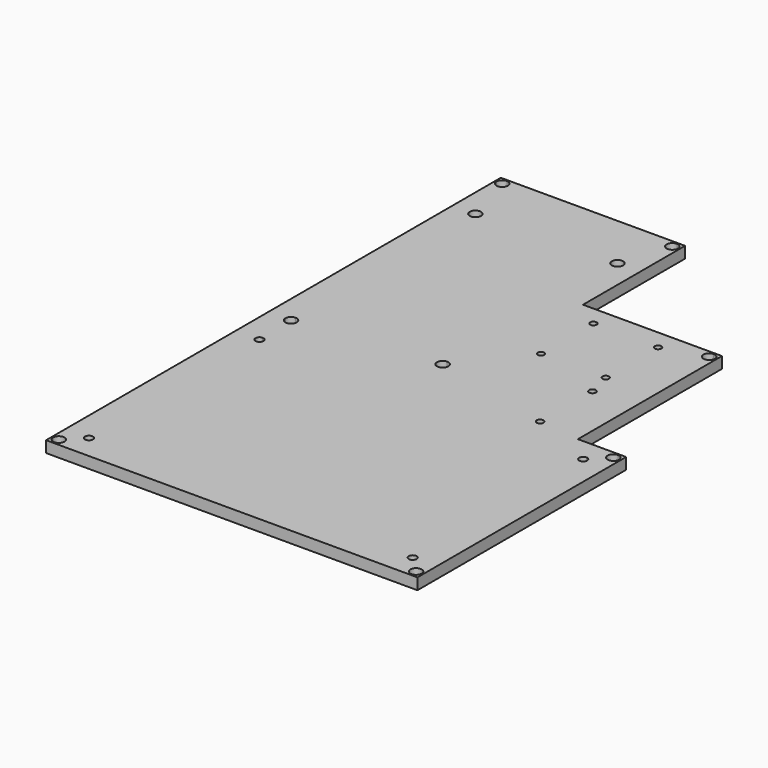
from build123d import *

# Parameters (mm, degrees)
F0_W     = 10
F0_H     = 17
F0_W_2   = 5
F0_H_2   = 5
F1_DEPTH = 4


with BuildPart() as f1:
    # F0 (on Top) → F1 (new body)
    with BuildSketch(Plane.XY):
        with BuildLine():
            Line((-37.7009056807, -58.8260023594), (-40.7009056807, -58.8260023594))
            Line((-40.7009056807, -58.8260023594), (-40.7009056807, -52.8260023594))
            Line((-40.7009056807, -52.8260023594), (-40.7009056807, 28.4739976406))
            Line((-40.7009056807, 28.4739976406), (-40.7009056807, 44.6739976406))
            Line((-40.7009056807, 44.6739976406), (14.2990943193, 44.6739976406))
            Line((14.2990943193, 44.6739976406), (14.2990943193, 49.6739976406))
            Line((14.2990943193, 49.6739976406), (-43.2009056807, 49.6739976406))
            Line((-43.2009056807, 49.6739976406), (-43.2009056807, 49.1739976406))
            ThreePointArc((-43.2009056807, 49.1739976406), (-41.7866921183, 48.588211203), (-41.2009056807, 47.1739976406))
            ThreePointArc((-41.2009056807, 47.1739976406), (-43.2009056807, 45.1739976406), (-45.2009056807, 47.1739976406))
            Line((-45.2009056807, 47.1739976406), (-45.7009056807, 47.1739976406))
            Line((-45.7009056807, 47.1739976406), (-45.7009056807, -148.3260023594))
            Line((-45.7009056807, -148.3260023594), (-45.2009056807, -148.3260023594))
            ThreePointArc((-45.2009056807, -148.3260023594), (-43.2009056807, -146.3260023594), (-41.2009056807, -148.3260023594))
            ThreePointArc((-41.2009056807, -148.3260023594), (-41.7866921183, -149.7402159218), (-43.2009056807, -150.3260023594))
            Line((-43.2009056807, -150.3260023594), (-43.2009056807, -150.8260023594))
            Line((-43.2009056807, -150.8260023594), (82.7990943193, -150.8260023594))
            Line((82.7990943193, -150.8260023594), (82.7990943193, -150.3260023594))
            ThreePointArc((82.7990943193, -150.3260023594), (81.384880757, -146.911788797), (84.7990943193, -148.3260023594))
            Line((84.7990943193, -148.3260023594), (85.2990943193, -148.3260023594))
            Line((85.2990943193, -148.3260023594), (85.2990943193, -63.8260023594))
            Line((85.2990943193, -63.8260023594), (80.2990943193, -63.8260023594))
            Line((80.2990943193, -63.8260023594), (80.2990943193, -58.8260023594))
            Line((80.2990943193, -58.8260023594), (68.2990943193, -58.8260023594))
            Line((68.2990943193, -58.8260023594), (68.2990943193, -22.3260023594))
            Line((68.2990943193, -22.3260023594), (68.2990943193, -5.3260023594))
            Line((68.2990943193, -5.3260023594), (63.2990943193, -5.3260023594))
            Line((63.2990943193, -5.3260023594), (63.2990943193, -22.3260023594))
            Line((63.2990943193, -22.3260023594), (53.2990943193, -22.3260023594))
            Line((53.2990943193, -22.3260023594), (53.2990943193, -25.3760023594))
            Line((53.2990943193, -25.3760023594), (53.2990943193, -27.3260023594))
            Line((53.2990943193, -27.3260023594), (51.3490943193, -27.3260023594))
            Line((51.3490943193, -27.3260023594), (28.5490943193, -27.3260023594))
            Line((28.5490943193, -27.3260023594), (19.2990943193, -27.3260023594))
            Line((19.2990943193, -27.3260023594), (19.2990943193, -25.3760023594))
            Line((19.2990943193, -25.3760023594), (19.2990943193, -2.2760023594))
            Line((19.2990943193, -2.2760023594), (19.2990943193, -0.3260023594))
            Line((19.2990943193, -0.3260023594), (14.2990943193, -0.3260023594))
            Line((14.2990943193, -0.3260023594), (14.2990943193, -27.3260023594))
            Line((14.2990943193, -27.3260023594), (14.2990943193, -32.3260023594))
            Line((14.2990943193, -32.3260023594), (14.2990943193, -47.2260023594))
            Line((14.2990943193, -47.2260023594), (14.2990943193, -58.8260023594))
            Line((14.2990943193, -58.8260023594), (11.2990943193, -58.8260023594))
            Line((11.2990943193, -58.8260023594), (-37.7009056807, -58.8260023594))
        make_face()
        Polygon((76.8990943193, -63.8260023594), (80.2990943193, -63.8260023594), (80.2990943193, -67.2260023594), (80.2990943193, -142.4260023594), (80.2990943193, -145.8260023594), (76.8990943193, -145.8260023594), (-37.3009056807, -145.8260023594), (-40.7009056807, -145.8260023594), (-40.7009056807, -142.4260023594), (-40.7009056807, -67.2260023594), (-40.7009056807, -63.8260023594), (-37.3009056807, -63.8260023594), (14.2990943193, -63.8260023594), (19.2990943193, -63.8260023594), align=None, mode=Mode.SUBTRACT)
        Polygon((53.5990943193, -58.8260023594), (19.2990943193, -58.8260023594), (19.2990943193, -32.3260023594), (53.5990943193, -32.3260023594), (55.2990943193, -32.3260023594), (55.2990943193, -34.0260023594), (55.2990943193, -57.1260023594), (55.2990943193, -58.8260023594), align=None, mode=Mode.SUBTRACT)
        with BuildLine():
            Line((76.8990943193, -65.8260023594), (76.8990943193, -63.8260023594))
            Line((76.8990943193, -63.8260023594), (19.2990943193, -63.8260023594))
            Line((19.2990943193, -63.8260023594), (14.2990943193, -63.8260023594))
            Line((14.2990943193, -63.8260023594), (-37.3009056807, -63.8260023594))
            Line((-37.3009056807, -63.8260023594), (-37.3009056807, -65.8260023594))
            ThreePointArc((-37.3009056807, -65.8260023594), (-36.310956187, -66.2360528657), (-35.9009056807, -67.2260023594))
            ThreePointArc((-35.9009056807, -67.2260023594), (-37.3009056807, -68.6260023594), (-38.7009056807, -67.2260023594))
            Line((-38.7009056807, -67.2260023594), (-40.7009056807, -67.2260023594))
            Line((-40.7009056807, -67.2260023594), (-40.7009056807, -142.4260023594))
            Line((-40.7009056807, -142.4260023594), (-38.7009056807, -142.4260023594))
            ThreePointArc((-38.7009056807, -142.4260023594), (-37.3009056807, -141.0260023594), (-35.9009056807, -142.4260023594))
            ThreePointArc((-35.9009056807, -142.4260023594), (-36.310956187, -143.4159518531), (-37.3009056807, -143.8260023594))
            Line((-37.3009056807, -143.8260023594), (-37.3009056807, -145.8260023594))
            Line((-37.3009056807, -145.8260023594), (76.8990943193, -145.8260023594))
            Line((76.8990943193, -145.8260023594), (76.8990943193, -143.8260023594))
            ThreePointArc((76.8990943193, -143.8260023594), (75.9091448257, -141.4360528657), (78.2990943193, -142.4260023594))
            Line((78.2990943193, -142.4260023594), (80.2990943193, -142.4260023594))
            Line((80.2990943193, -142.4260023594), (80.2990943193, -67.2260023594))
            Line((80.2990943193, -67.2260023594), (78.2990943193, -67.2260023594))
            ThreePointArc((78.2990943193, -67.2260023594), (75.9091448257, -68.2159518531), (76.8990943193, -65.8260023594))
        make_face()
        with BuildLine():
            Line((-37.7009056807, -54.8260023594), (-37.7009056807, -58.8260023594))
            Line((-37.7009056807, -58.8260023594), (11.2990943193, -58.8260023594))
            Line((11.2990943193, -58.8260023594), (11.2990943193, -49.2260023594))
            ThreePointArc((11.2990943193, -49.2260023594), (9.2990943193, -47.2260023594), (11.2990943193, -45.2260023594))
            Line((11.2990943193, -45.2260023594), (11.2990943193, 27.8739976406))
            ThreePointArc((11.2990943193, 27.8739976406), (9.884880757, 31.288211203), (13.2990943193, 29.8739976406))
            Line((13.2990943193, 29.8739976406), (14.2990943193, 29.8739976406))
            Line((14.2990943193, 29.8739976406), (14.2990943193, 44.6739976406))
            Line((14.2990943193, 44.6739976406), (-40.7009056807, 44.6739976406))
            Line((-40.7009056807, 44.6739976406), (-40.7009056807, 28.4739976406))
            Line((-40.7009056807, 28.4739976406), (-39.7009056807, 28.4739976406))
            ThreePointArc((-39.7009056807, 28.4739976406), (-37.7009056807, 30.4739976406), (-35.7009056807, 28.4739976406))
            ThreePointArc((-35.7009056807, 28.4739976406), (-36.2866921183, 27.0597840782), (-37.7009056807, 26.4739976406))
            Line((-37.7009056807, 26.4739976406), (-37.7009056807, -50.8260023594))
            ThreePointArc((-37.7009056807, -50.8260023594), (-36.2866921183, -51.411788797), (-35.7009056807, -52.8260023594))
            ThreePointArc((-35.7009056807, -52.8260023594), (-36.2866921183, -54.2402159218), (-37.7009056807, -54.8260023594))
        make_face()
        with BuildLine():
            Line((19.2990943193, -32.3260023594), (19.2990943193, -58.8260023594))
            Line((19.2990943193, -58.8260023594), (53.5990943193, -58.8260023594))
            Line((53.5990943193, -58.8260023594), (53.5990943193, -58.3260023594))
            ThreePointArc((53.5990943193, -58.3260023594), (52.7505661819, -56.277474222), (54.7990943193, -57.1260023594))
            Line((54.7990943193, -57.1260023594), (55.2990943193, -57.1260023594))
            Line((55.2990943193, -57.1260023594), (55.2990943193, -34.0260023594))
            Line((55.2990943193, -34.0260023594), (54.7990943193, -34.0260023594))
            ThreePointArc((54.7990943193, -34.0260023594), (52.7505661819, -34.8745304968), (53.5990943193, -32.8260023594))
            Line((53.5990943193, -32.8260023594), (53.5990943193, -32.3260023594))
            Line((53.5990943193, -32.3260023594), (19.2990943193, -32.3260023594))
        make_face()
        with BuildLine():
            Line((51.3490943193, -0.3260023594), (28.5490943193, -0.3260023594))
            Line((28.5490943193, -0.3260023594), (28.5490943193, -1.1260023594))
            ThreePointArc((28.5490943193, -1.1260023594), (29.3622671177, -1.462829561), (29.6990943193, -2.2760023594))
            ThreePointArc((29.6990943193, -2.2760023594), (28.5490943193, -3.4260023594), (27.3990943193, -2.2760023594))
            Line((27.3990943193, -2.2760023594), (19.2990943193, -2.2760023594))
            Line((19.2990943193, -2.2760023594), (19.2990943193, -25.3760023594))
            Line((19.2990943193, -25.3760023594), (27.3990943193, -25.3760023594))
            ThreePointArc((27.3990943193, -25.3760023594), (28.5490943193, -24.2260023594), (29.6990943193, -25.3760023594))
            ThreePointArc((29.6990943193, -25.3760023594), (29.3622671177, -26.1891751578), (28.5490943193, -26.5260023594))
            Line((28.5490943193, -26.5260023594), (28.5490943193, -27.3260023594))
            Line((28.5490943193, -27.3260023594), (51.3490943193, -27.3260023594))
            Line((51.3490943193, -27.3260023594), (51.3490943193, -26.5260023594))
            ThreePointArc((51.3490943193, -26.5260023594), (50.535921521, -24.562829561), (52.4990943193, -25.3760023594))
            Line((52.4990943193, -25.3760023594), (53.2990943193, -25.3760023594))
            Line((53.2990943193, -25.3760023594), (53.2990943193, -22.3260023594))
            Line((53.2990943193, -22.3260023594), (53.2990943193, -5.3260023594))
            Line((53.2990943193, -5.3260023594), (53.2990943193, -2.2760023594))
            Line((53.2990943193, -2.2760023594), (52.4990943193, -2.2760023594))
            ThreePointArc((52.4990943193, -2.2760023594), (50.535921521, -3.0891751578), (51.3490943193, -1.1260023594))
            Line((51.3490943193, -1.1260023594), (51.3490943193, -0.3260023594))
        make_face()
        with BuildLine():
            Line((65.7990943193, 4.6739976406), (19.2990943193, 4.6739976406))
            Line((19.2990943193, 4.6739976406), (19.2990943193, -0.3260023594))
            Line((19.2990943193, -0.3260023594), (28.5490943193, -0.3260023594))
            Line((28.5490943193, -0.3260023594), (51.3490943193, -0.3260023594))
            Line((51.3490943193, -0.3260023594), (53.2990943193, -0.3260023594))
            Line((53.2990943193, -0.3260023594), (53.2990943193, -2.2760023594))
            Line((53.2990943193, -2.2760023594), (53.2990943193, -5.3260023594))
            Line((53.2990943193, -5.3260023594), (63.2990943193, -5.3260023594))
            Line((63.2990943193, -5.3260023594), (68.2990943193, -5.3260023594))
            Line((68.2990943193, -5.3260023594), (68.2990943193, 2.1739976406))
            Line((68.2990943193, 2.1739976406), (67.7990943193, 2.1739976406))
            ThreePointArc((67.7990943193, 2.1739976406), (64.384880757, 0.7597840782), (65.7990943193, 4.1739976406))
            Line((65.7990943193, 4.1739976406), (65.7990943193, 4.6739976406))
        make_face()
        with BuildLine():
            Line((-40.7009056807, 28.4739976406), (-40.7009056807, -52.8260023594))
            Line((-40.7009056807, -52.8260023594), (-39.7009056807, -52.8260023594))
            ThreePointArc((-39.7009056807, -52.8260023594), (-39.115119243, -51.411788797), (-37.7009056807, -50.8260023594))
            Line((-37.7009056807, -50.8260023594), (-37.7009056807, 26.4739976406))
            ThreePointArc((-37.7009056807, 26.4739976406), (-39.115119243, 27.0597840782), (-39.7009056807, 28.4739976406))
            Line((-39.7009056807, 28.4739976406), (-40.7009056807, 28.4739976406))
        make_face()
        with BuildLine():
            Line((13.2990943193, -47.2260023594), (14.2990943193, -47.2260023594))
            Line((14.2990943193, -47.2260023594), (14.2990943193, -32.3260023594))
            Line((14.2990943193, -32.3260023594), (14.2990943193, -27.3260023594))
            Line((14.2990943193, -27.3260023594), (14.2990943193, -0.3260023594))
            Line((14.2990943193, -0.3260023594), (14.2990943193, 4.6739976406))
            Line((14.2990943193, 4.6739976406), (14.2990943193, 29.8739976406))
            Line((14.2990943193, 29.8739976406), (13.2990943193, 29.8739976406))
            ThreePointArc((13.2990943193, 29.8739976406), (12.7133078817, 28.4597840782), (11.2990943193, 27.8739976406))
            Line((11.2990943193, 27.8739976406), (11.2990943193, -45.2260023594))
            ThreePointArc((11.2990943193, -45.2260023594), (12.7133078817, -45.811788797), (13.2990943193, -47.2260023594))
        make_face()
        Polygon((16.7990943193, 44.6739976406), (14.2990943193, 44.6739976406), (14.2990943193, 29.8739976406), (14.2990943193, 4.6739976406), (19.2990943193, 4.6739976406), (19.2990943193, 44.6739976406), align=None)
        with Locations((58.2990943193, -13.8260023594)):
            Rectangle(F0_W, F0_H)
        with BuildLine():
            Line((11.2990943193, -49.2260023594), (11.2990943193, -58.8260023594))
            Line((11.2990943193, -58.8260023594), (14.2990943193, -58.8260023594))
            Line((14.2990943193, -58.8260023594), (14.2990943193, -47.2260023594))
            Line((14.2990943193, -47.2260023594), (13.2990943193, -47.2260023594))
            ThreePointArc((13.2990943193, -47.2260023594), (12.7133078817, -48.6402159218), (11.2990943193, -49.2260023594))
        make_face()
        with Locations((16.7990943193, 2.1739976406)):
            Rectangle(F0_W_2, F0_H_2)
        with BuildLine():
            Line((28.5490943193, -0.3260023594), (19.2990943193, -0.3260023594))
            Line((19.2990943193, -0.3260023594), (19.2990943193, -2.2760023594))
            Line((19.2990943193, -2.2760023594), (27.3990943193, -2.2760023594))
            ThreePointArc((27.3990943193, -2.2760023594), (27.735921521, -1.462829561), (28.5490943193, -1.1260023594))
            Line((28.5490943193, -1.1260023594), (28.5490943193, -0.3260023594))
        make_face()
        with BuildLine():
            Line((27.3990943193, -25.3760023594), (19.2990943193, -25.3760023594))
            Line((19.2990943193, -25.3760023594), (19.2990943193, -27.3260023594))
            Line((19.2990943193, -27.3260023594), (28.5490943193, -27.3260023594))
            Line((28.5490943193, -27.3260023594), (28.5490943193, -26.5260023594))
            ThreePointArc((28.5490943193, -26.5260023594), (27.735921521, -26.1891751578), (27.3990943193, -25.3760023594))
        make_face()
        with BuildLine():
            Line((-40.7009056807, -52.8260023594), (-40.7009056807, -58.8260023594))
            Line((-40.7009056807, -58.8260023594), (-37.7009056807, -58.8260023594))
            Line((-37.7009056807, -58.8260023594), (-37.7009056807, -54.8260023594))
            ThreePointArc((-37.7009056807, -54.8260023594), (-39.115119243, -54.2402159218), (-39.7009056807, -52.8260023594))
            Line((-39.7009056807, -52.8260023594), (-40.7009056807, -52.8260023594))
        make_face()
        with BuildLine():
            Line((80.2990943193, -67.2260023594), (80.2990943193, -63.8260023594))
            Line((80.2990943193, -63.8260023594), (76.8990943193, -63.8260023594))
            Line((76.8990943193, -63.8260023594), (76.8990943193, -65.8260023594))
            ThreePointArc((76.8990943193, -65.8260023594), (77.889043813, -66.2360528657), (78.2990943193, -67.2260023594))
            Line((78.2990943193, -67.2260023594), (80.2990943193, -67.2260023594))
        make_face()
        with BuildLine():
            Line((80.2990943193, -145.8260023594), (80.2990943193, -142.4260023594))
            Line((80.2990943193, -142.4260023594), (78.2990943193, -142.4260023594))
            ThreePointArc((78.2990943193, -142.4260023594), (77.889043813, -143.4159518531), (76.8990943193, -143.8260023594))
            Line((76.8990943193, -143.8260023594), (76.8990943193, -145.8260023594))
            Line((76.8990943193, -145.8260023594), (80.2990943193, -145.8260023594))
        make_face()
        with BuildLine():
            Line((-37.3009056807, -65.8260023594), (-37.3009056807, -63.8260023594))
            Line((-37.3009056807, -63.8260023594), (-40.7009056807, -63.8260023594))
            Line((-40.7009056807, -63.8260023594), (-40.7009056807, -67.2260023594))
            Line((-40.7009056807, -67.2260023594), (-38.7009056807, -67.2260023594))
            ThreePointArc((-38.7009056807, -67.2260023594), (-38.2908551743, -66.2360528657), (-37.3009056807, -65.8260023594))
        make_face()
        with BuildLine():
            Line((-40.7009056807, -145.8260023594), (-37.3009056807, -145.8260023594))
            Line((-37.3009056807, -145.8260023594), (-37.3009056807, -143.8260023594))
            ThreePointArc((-37.3009056807, -143.8260023594), (-38.2908551743, -143.4159518531), (-38.7009056807, -142.4260023594))
            Line((-38.7009056807, -142.4260023594), (-40.7009056807, -142.4260023594))
            Line((-40.7009056807, -142.4260023594), (-40.7009056807, -145.8260023594))
        make_face()
        with BuildLine():
            Line((14.2990943193, 49.6739976406), (14.2990943193, 44.6739976406))
            Line((14.2990943193, 44.6739976406), (16.7990943193, 44.6739976406))
            Line((16.7990943193, 44.6739976406), (19.2990943193, 44.6739976406))
            Line((19.2990943193, 44.6739976406), (19.2990943193, 47.1739976406))
            Line((19.2990943193, 47.1739976406), (18.7990943193, 47.1739976406))
            ThreePointArc((18.7990943193, 47.1739976406), (15.384880757, 45.7597840782), (16.7990943193, 49.1739976406))
            Line((16.7990943193, 49.1739976406), (16.7990943193, 49.6739976406))
            Line((16.7990943193, 49.6739976406), (14.2990943193, 49.6739976406))
        make_face()
        with BuildLine():
            Line((85.2990943193, -63.8260023594), (85.2990943193, -61.3260023594))
            Line((85.2990943193, -61.3260023594), (84.7990943193, -61.3260023594))
            ThreePointArc((84.7990943193, -61.3260023594), (81.384880757, -62.7402159218), (82.7990943193, -59.3260023594))
            Line((82.7990943193, -59.3260023594), (82.7990943193, -58.8260023594))
            Line((82.7990943193, -58.8260023594), (80.2990943193, -58.8260023594))
            Line((80.2990943193, -58.8260023594), (80.2990943193, -63.8260023594))
            Line((80.2990943193, -63.8260023594), (85.2990943193, -63.8260023594))
        make_face()
        with BuildLine():
            Line((-43.2009056807, 49.1739976406), (-43.2009056807, 49.6739976406))
            Line((-43.2009056807, 49.6739976406), (-45.7009056807, 49.6739976406))
            Line((-45.7009056807, 49.6739976406), (-45.7009056807, 47.1739976406))
            Line((-45.7009056807, 47.1739976406), (-45.2009056807, 47.1739976406))
            ThreePointArc((-45.2009056807, 47.1739976406), (-44.615119243, 48.588211203), (-43.2009056807, 49.1739976406))
        make_face()
        with BuildLine():
            Line((19.2990943193, 49.6739976406), (16.7990943193, 49.6739976406))
            Line((16.7990943193, 49.6739976406), (16.7990943193, 49.1739976406))
            ThreePointArc((16.7990943193, 49.1739976406), (18.2133078817, 48.588211203), (18.7990943193, 47.1739976406))
            Line((18.7990943193, 47.1739976406), (19.2990943193, 47.1739976406))
            Line((19.2990943193, 47.1739976406), (19.2990943193, 49.6739976406))
        make_face()
        with BuildLine():
            Line((68.2990943193, 4.6739976406), (65.7990943193, 4.6739976406))
            Line((65.7990943193, 4.6739976406), (65.7990943193, 4.1739976406))
            ThreePointArc((65.7990943193, 4.1739976406), (67.2133078817, 3.588211203), (67.7990943193, 2.1739976406))
            Line((67.7990943193, 2.1739976406), (68.2990943193, 2.1739976406))
            Line((68.2990943193, 2.1739976406), (68.2990943193, 4.6739976406))
        make_face()
        with BuildLine():
            Line((-45.2009056807, -148.3260023594), (-45.7009056807, -148.3260023594))
            Line((-45.7009056807, -148.3260023594), (-45.7009056807, -150.8260023594))
            Line((-45.7009056807, -150.8260023594), (-43.2009056807, -150.8260023594))
            Line((-43.2009056807, -150.8260023594), (-43.2009056807, -150.3260023594))
            ThreePointArc((-43.2009056807, -150.3260023594), (-44.615119243, -149.7402159218), (-45.2009056807, -148.3260023594))
        make_face()
        with BuildLine():
            Line((82.7990943193, -150.3260023594), (82.7990943193, -150.8260023594))
            Line((82.7990943193, -150.8260023594), (85.2990943193, -150.8260023594))
            Line((85.2990943193, -150.8260023594), (85.2990943193, -148.3260023594))
            Line((85.2990943193, -148.3260023594), (84.7990943193, -148.3260023594))
            ThreePointArc((84.7990943193, -148.3260023594), (84.2133078817, -149.7402159218), (82.7990943193, -150.3260023594))
        make_face()
        with BuildLine():
            Line((85.2990943193, -61.3260023594), (85.2990943193, -58.8260023594))
            Line((85.2990943193, -58.8260023594), (82.7990943193, -58.8260023594))
            Line((82.7990943193, -58.8260023594), (82.7990943193, -59.3260023594))
            ThreePointArc((82.7990943193, -59.3260023594), (84.2133078817, -59.911788797), (84.7990943193, -61.3260023594))
            Line((84.7990943193, -61.3260023594), (85.2990943193, -61.3260023594))
        make_face()
        with BuildLine():
            Line((53.2990943193, -0.3260023594), (51.3490943193, -0.3260023594))
            Line((51.3490943193, -0.3260023594), (51.3490943193, -1.1260023594))
            ThreePointArc((51.3490943193, -1.1260023594), (52.1622671177, -1.462829561), (52.4990943193, -2.2760023594))
            Line((52.4990943193, -2.2760023594), (53.2990943193, -2.2760023594))
            Line((53.2990943193, -2.2760023594), (53.2990943193, -0.3260023594))
        make_face()
        with BuildLine():
            Line((51.3490943193, -26.5260023594), (51.3490943193, -27.3260023594))
            Line((51.3490943193, -27.3260023594), (53.2990943193, -27.3260023594))
            Line((53.2990943193, -27.3260023594), (53.2990943193, -25.3760023594))
            Line((53.2990943193, -25.3760023594), (52.4990943193, -25.3760023594))
            ThreePointArc((52.4990943193, -25.3760023594), (52.1622671177, -26.1891751578), (51.3490943193, -26.5260023594))
        make_face()
        with BuildLine():
            Line((53.5990943193, -58.3260023594), (53.5990943193, -58.8260023594))
            Line((53.5990943193, -58.8260023594), (55.2990943193, -58.8260023594))
            Line((55.2990943193, -58.8260023594), (55.2990943193, -57.1260023594))
            Line((55.2990943193, -57.1260023594), (54.7990943193, -57.1260023594))
            ThreePointArc((54.7990943193, -57.1260023594), (54.4476224568, -57.9745304968), (53.5990943193, -58.3260023594))
        make_face()
        with BuildLine():
            Line((55.2990943193, -32.3260023594), (53.5990943193, -32.3260023594))
            Line((53.5990943193, -32.3260023594), (53.5990943193, -32.8260023594))
            ThreePointArc((53.5990943193, -32.8260023594), (54.4476224568, -33.177474222), (54.7990943193, -34.0260023594))
            Line((54.7990943193, -34.0260023594), (55.2990943193, -34.0260023594))
            Line((55.2990943193, -34.0260023594), (55.2990943193, -32.3260023594))
        make_face()
    extrude(amount=F1_DEPTH)


solid = f1.part
